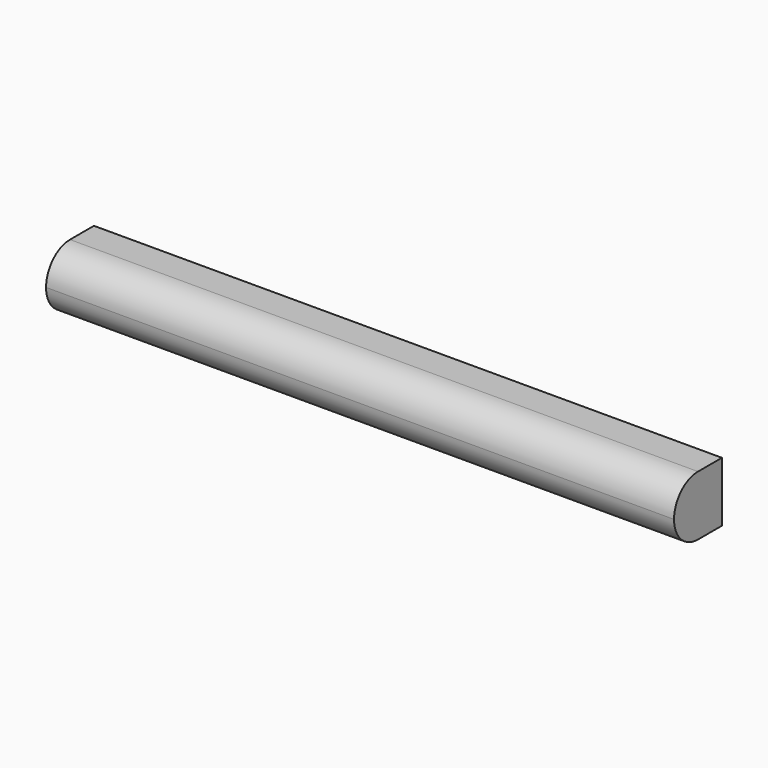
from build123d import *

# Parameters (mm, degrees)
F0_W     = 105
F0_H     = 10
F1_DEPTH = 10
F2_R     = 4.99999


# Not quite as in the source:
# - a fillet or chamfer is up to 0.001 mm smaller than in the source, because OpenCascade refuses the exact size


with BuildPart() as f1:
    # F0 (on Front) → F1 (new body)
    with BuildSketch(Plane.XZ):
        Rectangle(F0_W, F0_H)
    extrude(amount=F1_DEPTH)

    # F2 (radius 5 in the source; OpenCascade refuses exactly that, so slightly less here)
    f2_edges = [f1.edges().sort_by_distance(p)[0] for p in [
        (0, -10, -5),
        (0, -10, 5),
    ]]
    fillet(f2_edges, radius=F2_R)


solid = f1.part
